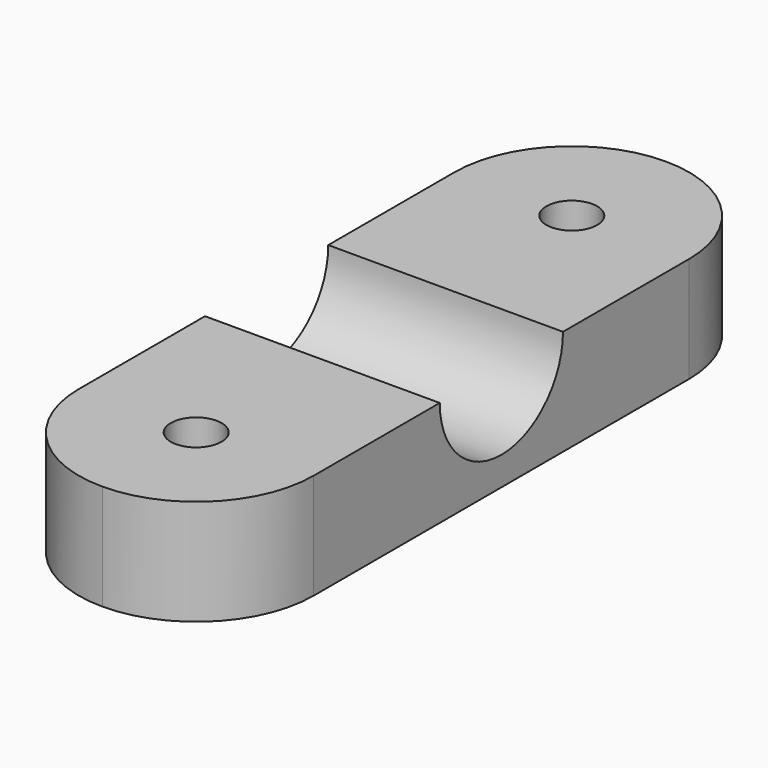
from build123d import *

# Parameters (mm, degrees)
F0_W          = 25.4
F0_H          = 76.2
F1_DEPTH      = 11.43
F3_DEPTH      = 12.701
F3_DEPTH_BACK = 12.701
F5_D          = 5.5
F6_R          = 12.69999


# Not quite as in the source:
# - a fillet or chamfer is up to 0.001 mm smaller than in the source, because OpenCascade refuses the exact size
# - a pattern or mirror of a feature is missing from the dataset's text; its kind, count and spacing are read off the source's solid


with BuildPart() as f1:
    # F0 (on Top) → F1 (new body)
    with BuildSketch(Plane.XY):
        Rectangle(F0_W, F0_H)
    extrude(amount=F1_DEPTH)

    # F2 (on Right) → F3 (cut, two sides)
    with BuildSketch(Plane.YZ) as f3_sk:
        with BuildLine():
            Line((8.334375, 11.43), (-8.334375, 11.43))
            ThreePointArc((-8.334375, 11.43), (0, 3.095625), (8.334375, 11.43))
        make_face()
    extrude(amount=-F3_DEPTH, mode=Mode.SUBTRACT)
    extrude(f3_sk.sketch, amount=F3_DEPTH_BACK, mode=Mode.SUBTRACT)

    # F5 (through all)
    with Locations(Plane(origin=(0, 0, 0), x_dir=(1, 0, 0), z_dir=(0, 0, -1))):
        with Locations((0, 25.4)):
            f5 = Hole(F5_D / 2)

    # F5_copies: F5 across plane
    add(f5.mirror(Plane.ZX), mode=Mode.SUBTRACT)

    # F6 (radius 12.7 in the source; OpenCascade refuses exactly that, so slightly less here)
    f6_edges = [f1.edges().sort_by_distance(p)[0] for p in [
        (-12.7, -38.1, 5.715),
        (12.7, -38.1, 5.715),
        (-12.7, 38.1, 5.715),
        (12.7, 38.1, 5.715),
    ]]
    fillet(f6_edges, radius=F6_R)


solid = f1.part
